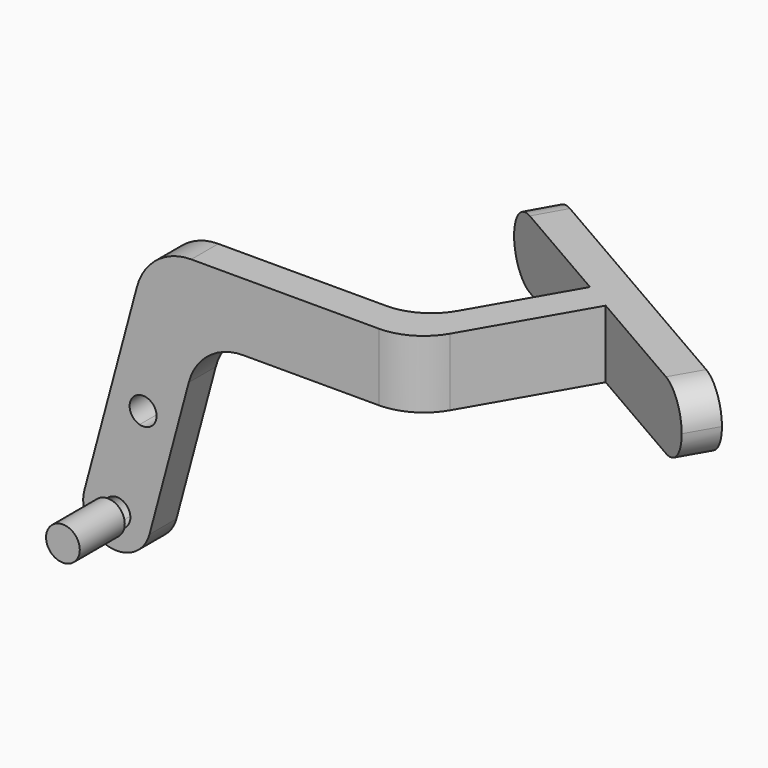
from build123d import *

# Parameters (mm, degrees)
F3_R     = 1.5
F4_DEPTH = 5
F5_DEPTH = 100
F0_W     = 123.8063722849
F0_H     = 159.0860895813
F6_DEPTH = 31.2010005245
F7_R     = 2.99999


# Not quite as in the source:
# - a fillet or chamfer is up to 0.001 mm smaller than in the source, because OpenCascade refuses the exact size


with BuildPart() as f4:
    # F3 (on offset) → F4 (new body)
    with BuildSketch(Plane.XZ.offset(1)):
        with Locations((0, -28.2000005245)):
            Circle(F3_R)
    extrude(amount=F4_DEPTH)


with BuildPart() as f5:
    # F1 (on Front) → F5 (new body)
    with BuildSketch(Plane.XZ):
        with BuildLine():
            Line((1.7853418934, -9.9459039539), (-2.8977774789, -27.4235433892))
            ThreePointArc((-2.8977774789, -27.4235433892), (-2.5980762114, -29.7000005245), (-0.7764571353, -31.0977780034))
            ThreePointArc((-0.7764571353, -31.0977780034), (1.5, -30.7980767359), (2.8977774789, -28.9764576598))
            Line((2.8977774789, -28.9764576598), (6.3893038213, -15.9459039539))
            ThreePointArc((6.3893038213, -15.9459039539), (8.1751258077, -13.273232478), (11.2189329527, -12.2399991794))
            Line((11.2189329527, -12.2399991794), (56.5063462641, -12.2399991794))
            Line((56.5063462641, -12.2399991794), (56.5063462641, -6.2399991794))
            Line((56.5063462641, -6.2399991794), (6.6149710249, -6.2399991794))
            ThreePointArc((6.6149710249, -6.2399991794), (3.5711638798, -7.273232478), (1.7853418934, -9.9459039539))
        make_face()
        with BuildLine():
            ThreePointArc((1.2, -28.2000005245), (0.7305137148, -29.1520245329), (-0.3105828541, -29.3591115161))
            ThreePointArc((-0.3105828541, -29.3591115161), (-1.1591109915, -27.8894176704), (0.3105828541, -27.040889533))
            ThreePointArc((0.3105828541, -27.040889533), (0.9520240083, -27.4694868097), (1.2, -28.2000005245))
        make_face(mode=Mode.SUBTRACT)
        with BuildLine():
            ThreePointArc((3.5293714059, -19.5066680879), (3.0598851207, -20.4586920963), (2.0187885518, -20.6657790795))
            ThreePointArc((2.0187885518, -20.6657790795), (1.5988576911, -18.5546440796), (3.5293714059, -19.5066680879))
        make_face(mode=Mode.SUBTRACT)
    extrude(amount=-F5_DEPTH)

    # F0 (on Top) → F6 (cut, through all)
    with BuildSketch(Plane.XY):
        with Locations((20.0330018997, 51.0744024068)):
            Rectangle(F0_W, F0_H)
        with BuildLine():
            Line((30.8290268609, 14.0490771528), (18.2928432391, 21.2868461414))
            Line((18.2928432391, 21.2868461414), (19.771658506, 23.8971533641))
            Line((19.771658506, 23.8971533641), (47.4844714271, 7.8971533641))
            Line((47.4844714271, 7.8971533641), (45.9844714271, 5.2990771528))
            Line((45.9844714271, 5.2990771528), (33.4271030722, 12.5490771528))
            Line((33.4271030722, 12.5490771528), (27.625265673, 2.5))
            ThreePointArc((27.625265673, 2.5), (25.7951386541, 0.6698729811), (23.2951386541, 0))
            Line((23.2951386541, 0), (0, 0))
            Line((0, 0), (-9.2670181766, 0))
            Line((-9.2670181766, 0), (-9.2670181766, 3))
            Line((-9.2670181766, 3), (0, 3))
            Line((0, 3), (21.5630878465, 3))
            ThreePointArc((21.5630878465, 3), (24.0630878465, 3.6698729811), (25.8932148654, 5.5))
            Line((25.8932148654, 5.5), (30.8290268609, 14.0490771528))
        make_face(mode=Mode.SUBTRACT)
        with BuildLine():
            ThreePointArc((186.4293499082, 37.2767830718), (189.1206068421, 41.7118372377), (194.29723209, 41.3725432932))
            Line((194.29723209, 41.3725432932), (212.3185770643, 28.7538616935))
            Line((212.3185770643, 28.7538616935), (214.0393063734, 31.2113178264))
            Line((214.0393063734, 31.2113178264), (196.017961399, 43.8299994261))
            ThreePointArc((196.017961399, 43.8299994261), (187.7353610024, 44.3728697372), (183.4293499082, 37.2767830718))
            Line((183.4293499082, 37.2767830718), (183.4293499082, 8.5356936807))
            ThreePointArc((183.4293499082, 8.5356936807), (181.9648838142, 5.0001597747), (178.4293499082, 3.5356936807))
            Line((178.4293499082, 3.5356936807), (134.4964219123, 3.5356936807))
            Line((134.4964219123, 3.5356936807), (134.4964219123, 0.5356936807))
            Line((134.4964219123, 0.5356936807), (178.4293499082, 0.5356936807))
            ThreePointArc((178.4293499082, 0.5356936807), (184.0862041577, 2.8788394312), (186.4293499082, 8.5356936807))
            Line((186.4293499082, 8.5356936807), (186.4293499082, 37.2767830718))
        make_face()
    extrude(amount=-F6_DEPTH, mode=Mode.SUBTRACT)

    # F7 (radius 3 in the source; OpenCascade refuses exactly that, so slightly less here)
    f7_edges = [f5.edges().sort_by_distance(p)[0] for p in [
        (19.032251, 22.592, -6.239999),
        (46.734471, 6.598115, -6.239999),
        (46.734471, 6.598115, -12.239999),
        (19.032251, 22.592, -12.239999),
    ]]
    fillet(f7_edges, radius=F7_R)


solid = Compound([f4.part, f5.part])
